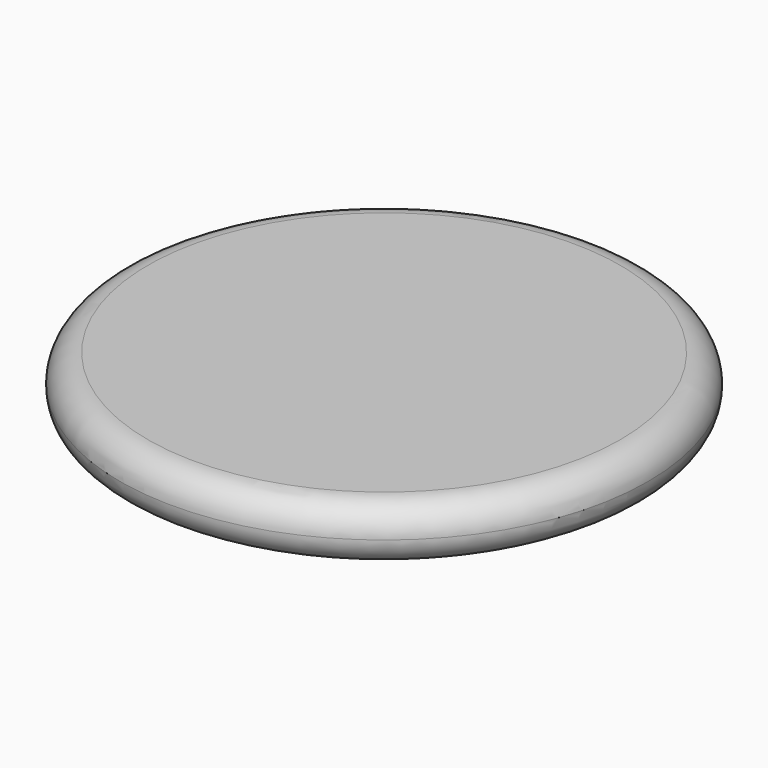
from build123d import *

# Parameters (mm, degrees)
F0_R     = 47.5522600406
F1_DEPTH = 10
F2_R     = 5
F3_R     = 4.99999


# Not quite as in the source:
# - a fillet or chamfer is up to 0.001 mm smaller than in the source, because OpenCascade refuses the exact size


with BuildPart() as f1:
    # F0 (on Top) → F1 (new body)
    with BuildSketch(Plane.XY):
        Circle(F0_R)
    extrude(amount=F1_DEPTH)

    # F2
    f2_edges = [f1.edges().sort_by_distance(p)[0] for p in [
        (-47.55226, 0, 10),
    ]]
    fillet(f2_edges, radius=F2_R)

    # F3 (radius 5 in the source; OpenCascade refuses exactly that, so slightly less here)
    f3_edges = [f1.edges().sort_by_distance(p)[0] for p in [
        (-47.55226, 0, 0),
    ]]
    fillet(f3_edges, radius=F3_R)


solid = f1.part
